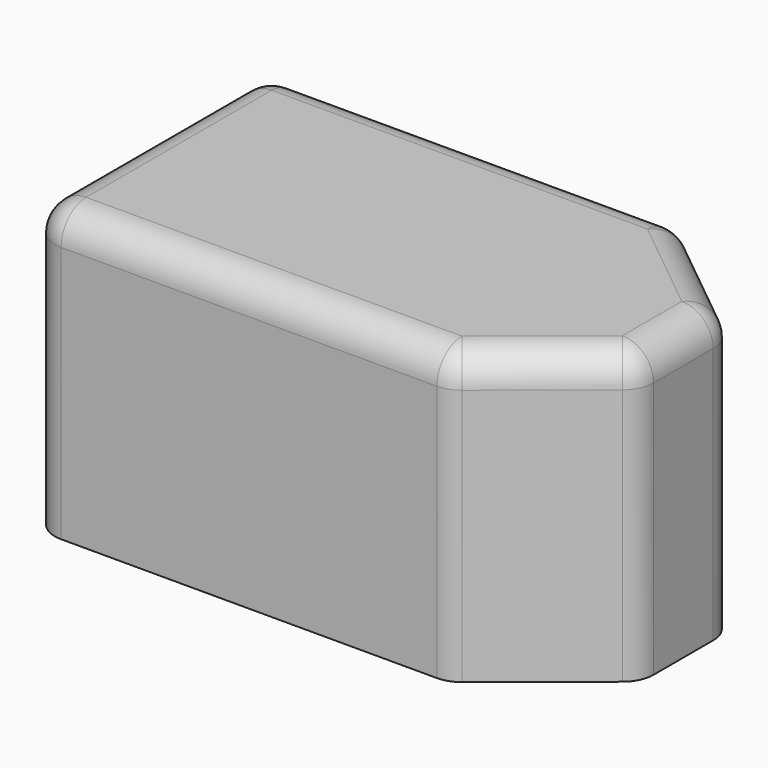
from build123d import *

# Parameters (mm, degrees)
F1_DEPTH = 8.3
F3_DEPTH = 8.2
F5_DEPTH = 1
F6_R     = 1
F7_SIZE  = 0.75


with BuildPart() as f1:
    # F0 (on Top) → F1 (new body)
    with BuildSketch(Plane.XY):
        Polygon((0, 6.3), (0, 0), (11.25, 0), (14, 2.225), (14, 4.075), (11.25, 6.3), align=None)
    extrude(amount=F1_DEPTH)


with BuildPart() as f3:
    # F2 (on face) → F3 (new body)
    with BuildSketch(Plane.XY.offset(8.3)):
        Polygon((-1.55, 7.85), (-1.55, -1.55), (11.7985185798, -1.55), (15.55, 1.4852895127), (15.55, 4.8147104873), (11.7985185798, 7.85), align=None)
        Polygon((11.2676941477, -0.05), (-0.05, -0.05), (-0.05, 6.35), (11.2676941477, 6.35), (14.05, 4.0988616286), (14.05, 2.2011383714), align=None, mode=Mode.SUBTRACT)
    extrude(amount=-F3_DEPTH)

    # F4 (on face) → F5 (join)
    with BuildSketch(Plane.XY.offset(8.3)):
        Polygon((11.7985185798, 7.85), (-1.55, 7.85), (-1.55, -1.55), (11.7985185798, -1.55), (15.55, 1.4852895127), (15.55, 4.8147104873), align=None)
    extrude(amount=F5_DEPTH)

    # F6
    f6_edges = [f3.edges().sort_by_distance(p)[0] for p in [
        (5.124259, 7.85, 9.3),
        (-1.55, 3.15, 9.3),
        (5.124259, -1.55, 9.3),
        (13.674259, -0.032355, 9.3),
        (15.55, 3.15, 9.3),
        (13.674259, 6.332355, 9.3),
        (-1.55, -1.55, 4.7),
        (-1.55, 7.85, 4.7),
        (11.798519, 7.85, 4.7),
        (15.55, 4.81471, 4.7),
        (15.55, 1.48529, 4.7),
        (11.798519, -1.55, 4.7),
    ]]
    fillet(f6_edges, radius=F6_R)

    # F7
    f7_edges = [f3.edges().sort_by_distance(p)[0] for p in [
        (12.658847, 1.075569, 0.1),
        (14.05, 3.15, 0.1),
        (12.658847, 5.224431, 0.1),
        (5.608847, 6.35, 0.1),
        (-0.05, 3.15, 0.1),
        (5.608847, -0.05, 0.1),
    ]]
    chamfer(f7_edges, length=F7_SIZE)


solid = Compound([f1.part, f3.part])
